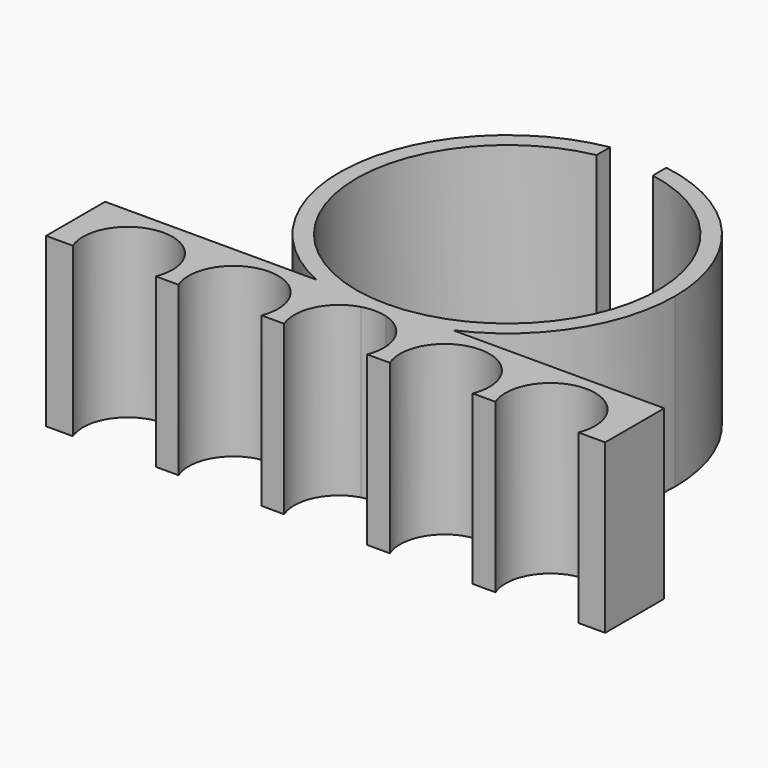
from build123d import *

# Parameters (mm, degrees)
F0_R     = 17.145
F1_DEPTH = 19.05
F2_DEPTH = 25.4
F3_W     = 6.35
F3_H     = 30.0934736039
F4_DEPTH = 25.4


# Not quite as in the source:
# - a feature names something its author has since deleted; it is built from what else it names


with BuildPart() as f1:
    # F0 (on Top) → F1 (new body)
    with BuildSketch(Plane.XY):
        with BuildLine():
            ThreePointArc((7.7574028515, -17.399), (15.9793777151, -10.3712095649), (19.05, 0))
            ThreePointArc((19.05, 0), (-10.3712095649, 15.9793777151), (-7.7574028515, -17.399))
            Line((-7.7574028515, -17.399), (7.7574028515, -17.399))
        make_face()
        Circle(F0_R, mode=Mode.SUBTRACT)
        with BuildLine():
            Line((7.7574028515, -17.399), (-7.7574028515, -17.399))
            ThreePointArc((-7.7574028515, -17.399), (-4.6557505543, -18.472316768), (-1.4158987787, -18.9973085106))
            ThreePointArc((-1.4158987787, -18.9973085106), (0, -18.796), (1.4158987787, -18.9973085106))
            ThreePointArc((1.4158987787, -18.9973085106), (4.6557505543, -18.472316768), (7.7574028515, -17.399))
        make_face()
        with BuildLine():
            Line((31.75, -17.399), (7.7574028515, -17.399))
            ThreePointArc((7.7574028515, -17.399), (4.6557505543, -18.472316768), (1.4158987787, -18.9973085106))
            ThreePointArc((1.4158987787, -18.9973085106), (4.0619678603, -20.8252923605), (5.08, -23.876))
            ThreePointArc((5.08, -23.876), (4.9864603217, -24.8463676933), (4.7092860393, -25.781))
            Line((4.7092860393, -25.781), (7.2907139607, -25.781))
            ThreePointArc((7.2907139607, -25.781), (11.0296323067, -18.8895396783), (17.08, -23.876))
            ThreePointArc((17.08, -23.876), (16.9864603217, -24.8463676933), (16.7092860393, -25.781))
            Line((16.7092860393, -25.781), (19.2907139607, -25.781))
            ThreePointArc((19.2907139607, -25.781), (23.0296323067, -18.8895396783), (29.08, -23.876))
            ThreePointArc((29.08, -23.876), (28.9864603217, -24.8463676933), (28.7092860393, -25.781))
            Line((28.7092860393, -25.781), (31.75, -25.781))
            Line((31.75, -25.781), (31.75, -17.399))
        make_face()
        with BuildLine():
            ThreePointArc((-1.4158987787, -18.9973085106), (-4.6557505543, -18.472316768), (-7.7574028515, -17.399))
            Line((-7.7574028515, -17.399), (-31.75, -17.399))
            Line((-31.75, -17.399), (-31.75, -25.781))
            Line((-31.75, -25.781), (-28.7092860393, -25.781))
            ThreePointArc((-28.7092860393, -25.781), (-24.9703676933, -18.8895396783), (-18.92, -23.876))
            ThreePointArc((-18.92, -23.876), (-19.0135396783, -24.8463676933), (-19.2907139607, -25.781))
            Line((-19.2907139607, -25.781), (-16.7092860393, -25.781))
            ThreePointArc((-16.7092860393, -25.781), (-12.9703676933, -18.8895396783), (-6.92, -23.876))
            ThreePointArc((-6.92, -23.876), (-7.0135396783, -24.8463676933), (-7.2907139607, -25.781))
            Line((-7.2907139607, -25.781), (-4.7092860393, -25.781))
            ThreePointArc((-4.7092860393, -25.781), (-4.5699113579, -21.6573720049), (-1.4158987787, -18.9973085106))
        make_face()
    extrude(amount=F1_DEPTH)

    # F0 (on Top) → F2 (cut)
    with BuildSketch(Plane.XY):
        with BuildLine():
            Line((-16.7092860393, -25.781), (-7.2907139607, -25.781))
            ThreePointArc((-7.2907139607, -25.781), (-7.0135396783, -24.8463676933), (-6.92, -23.876))
            ThreePointArc((-6.92, -23.876), (-12.9703676933, -18.8895396783), (-16.7092860393, -25.781))
        make_face()
        with BuildLine():
            ThreePointArc((-18.92, -23.876), (-24.9703676933, -18.8895396783), (-28.7092860393, -25.781))
            Line((-28.7092860393, -25.781), (-19.2907139607, -25.781))
            ThreePointArc((-19.2907139607, -25.781), (-19.0135396783, -24.8463676933), (-18.92, -23.876))
        make_face()
        with BuildLine():
            ThreePointArc((17.08, -23.876), (11.0296323067, -18.8895396783), (7.2907139607, -25.781))
            Line((7.2907139607, -25.781), (16.7092860393, -25.781))
            ThreePointArc((16.7092860393, -25.781), (16.9864603217, -24.8463676933), (17.08, -23.876))
        make_face()
    extrude(amount=F2_DEPTH, mode=Mode.SUBTRACT)

    # F3 (on Top) → F4 (cut)
    with BuildSketch(Plane.XY):
        with Locations((-0.1380435133, 15.0467368019)):
            Rectangle(F3_W, F3_H)
    extrude(amount=F4_DEPTH, mode=Mode.SUBTRACT)


solid = f1.part
